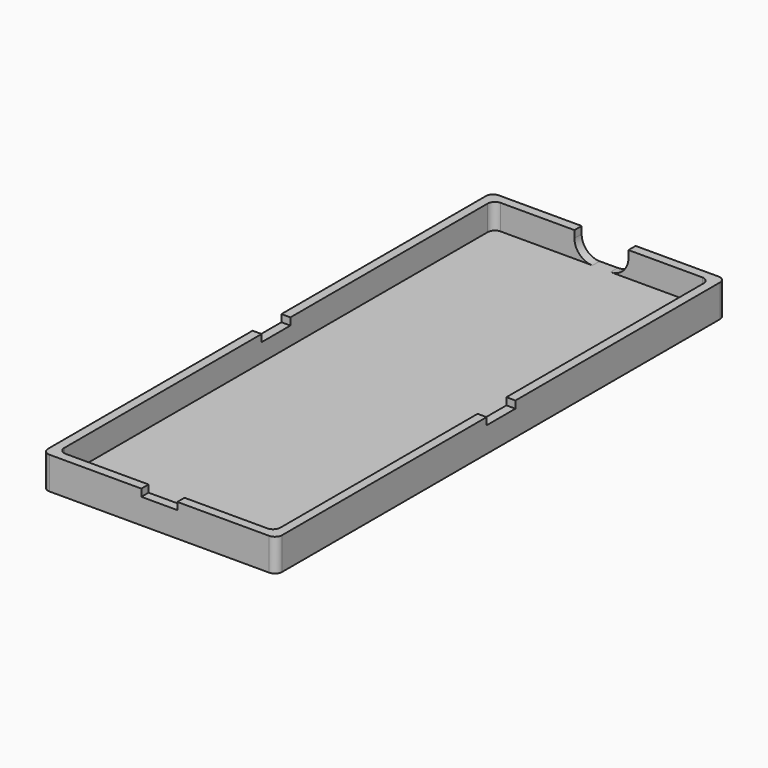
from build123d import *

# Parameters (mm, degrees)
F0_W      = 65
F0_H      = 156
F0_W_2    = 60
F0_H_2    = 151
F1_DEPTH  = 2
F2_DEPTH  = 7
F3_W      = 10
F3_H      = 2.5
F4_DEPTH  = 5
F5_DEPTH  = 2
F6_R      = 2
F7_R      = 2
F8_W      = 5
F8_H      = 2.5
F8_W_2    = 2.5
F8_H_2    = 5
F9_DEPTH  = 2
F10_DEPTH = 2.5
F11_DEPTH = 2.5
F12_R     = 5


with BuildPart() as f1:
    # F0 (on Top) → F1 (new body)
    with BuildSketch(Plane.XY):
        Rectangle(F0_W, F0_H)
        Rectangle(F0_W_2, F0_H_2, mode=Mode.SUBTRACT)
        Rectangle(F0_W_2, F0_H_2)
    extrude(amount=F1_DEPTH)

    # F0 (on Top) → F2 (join)
    with BuildSketch(Plane.XY):
        Rectangle(F0_W, F0_H)
        Rectangle(F0_W_2, F0_H_2, mode=Mode.SUBTRACT)
    extrude(amount=F2_DEPTH)

    # F3 (on face) → F4 (cut, through all)
    with BuildSketch(Plane.XY.offset(7)):
        with Locations((5, 76.75)):
            Rectangle(F3_W, F3_H)
        with Locations((-5, 76.75)):
            Rectangle(F3_W, F3_H)
    extrude(amount=-F4_DEPTH, mode=Mode.SUBTRACT)

    # F5 (add): a face of the model
    f5_faces = [f1.faces().sort_by_distance(p)[0] for p in [
        (0, -76.31, 7),
    ]]
    extrude(f5_faces, amount=F5_DEPTH)

    # F6
    f6_edges = [f1.edges().sort_by_distance(p)[0] for p in [
        (-32.5, 78, 4.5),
        (32.5, 78, 4.5),
        (32.5, -78, 4.5),
        (-32.5, -78, 4.5),
    ]]
    fillet(f6_edges, radius=F6_R)

    # F7
    f7_edges = [f1.edges().sort_by_distance(p)[0] for p in [
        (-30, 75.5, 5.5),
        (30, 75.5, 5.5),
        (30, -75.5, 5.5),
        (-30, -75.5, 5.5),
    ]]
    fillet(f7_edges, radius=F7_R)

    # F8 (on face) → F9 (cut)
    with BuildSketch(Plane.XY.offset(9)):
        with Locations((2.5, -76.75)):
            Rectangle(F8_W, F8_H)
        with Locations((-2.5, -76.75)):
            Rectangle(F8_W, F8_H)
        with Locations((-31.25, 2.5)):
            Rectangle(F8_W_2, F8_H_2)
        with Locations((-31.25, -2.5)):
            Rectangle(F8_W_2, F8_H_2)
        with Locations((31.25, 2.5)):
            Rectangle(F8_W_2, F8_H_2)
        with Locations((31.25, -2.5)):
            Rectangle(F8_W_2, F8_H_2)
    extrude(amount=-F9_DEPTH, mode=Mode.SUBTRACT)

    # F10 (add): a face of the model
    f10_faces = [f1.faces().sort_by_distance(p)[0] for p in [
        (-10, 76.75, 5.5),
    ]]
    extrude(f10_faces, amount=F10_DEPTH)

    # F11 (add): a face of the model
    f11_faces = [f1.faces().sort_by_distance(p)[0] for p in [
        (10, 76.75, 5.5),
    ]]
    extrude(f11_faces, amount=F11_DEPTH)

    # F12
    f12_edges = [f1.edges().sort_by_distance(p)[0] for p in [
        (7.5, 76.75, 2),
        (-7.5, 76.75, 2),
    ]]
    fillet(f12_edges, radius=F12_R)


solid = f1.part
